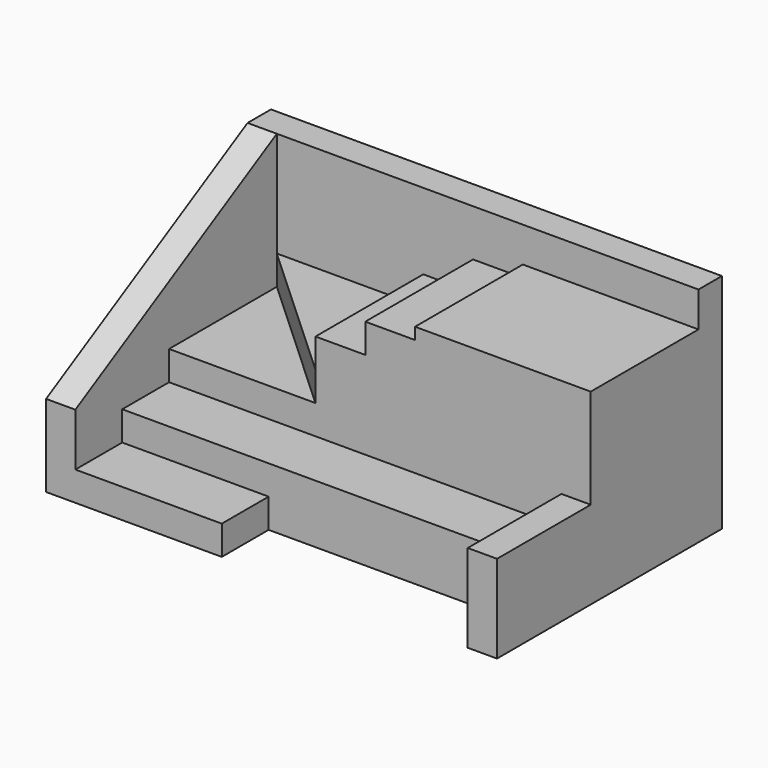
from build123d import *

# Parameters (mm, degrees)
F1_DEPTH  = 38
F3_DEPTH  = 25
F4_DEPTH  = 38
F0_W      = 25
F0_H      = 10
F5_DEPTH  = 5
F6_DEPTH  = 10
F7_DEPTH  = 15
F0_W_2    = 5
F0_H_2    = 5
F8_DEPTH  = 38
F0_H_3    = 23
F9_DEPTH  = 32
F11_DEPTH = 15
F12_DEPTH = 20
F0_W_3    = 8.5
F13_DEPTH = 25
F14_DEPTH = 30
F15_DEPTH = 32


# Not quite as in the source:
# - the program builds the solid bodies; features that only make, move or delete a surface that nothing else refers to are left out


with BuildPart() as f1:
    # F0 (on Top) → F1 (new body)
    with BuildSketch(Plane.XY):
        Polygon((-33.5, 19), (-38.5, 19), (-38.5, -24), (-33.5, -24), (-33.5, -14), (-33.5, -4), align=None)
    extrude(amount=F1_DEPTH)

    # F2 (on face) → F3 (cut)
    with BuildSketch(Plane.YZ.offset(-33.5)):
        Polygon((-24, 38), (-24, 14), (19, 38), align=None)
    extrude(amount=-F3_DEPTH, mode=Mode.SUBTRACT)

    # F0 (on Top) → F4 (join)
    with BuildSketch(Plane.XY):
        Polygon((33.5, 19), (33.5, 24), (-38.5, 24), (-38.5, 19), (-33.5, 19), (-8.5, 19), (0, 19), (8.5, 19), align=None)
    extrude(amount=F4_DEPTH)

    # F0 (on Top) → F5 (join)
    with BuildSketch(Plane.XY):
        with Locations((-21, -19)):
            Rectangle(F0_W, F0_H)
    extrude(amount=F5_DEPTH)

    # F0 (on Top) → F6 (join)
    with BuildSketch(Plane.XY):
        Polygon((33.5, -14), (33.5, -4), (8.5, -4), (0, -4), (-8.5, -4), (-33.5, -4), (-33.5, -14), (-8.5, -14), align=None)
    extrude(amount=F6_DEPTH)

    # F0 (on Top) → F7 (join)
    with BuildSketch(Plane.XY):
        Polygon((38.5, -24), (38.5, -4), (33.5, -4), (33.5, -14), (33.5, -24), align=None)
    extrude(amount=F7_DEPTH)

    # F0 (on Top) → F8 (join)
    with BuildSketch(Plane.XY):
        with Locations((36, 21.5)):
            Rectangle(F0_W_2, F0_H_2)
    extrude(amount=F8_DEPTH)

    # F0 (on Top) → F9 (join)
    with BuildSketch(Plane.XY):
        with Locations((36, 7.5)):
            Rectangle(F0_W_2, F0_H_3)
    extrude(amount=F9_DEPTH)

    # F0 (on Top) → F11 (join)
    with BuildSketch(Plane.XY):
        Polygon((-8.5, -4), (-33.5, 19), (-33.5, -4), align=None)
    extrude(amount=F11_DEPTH)

    # F0 (on Top) → F12 (join)
    with BuildSketch(Plane.XY):
        Polygon((-8.5, 19), (-33.5, 19), (-8.5, -4), align=None)
    extrude(amount=F12_DEPTH)

    # F0 (on Top) → F13 (join)
    with BuildSketch(Plane.XY):
        with Locations((-4.25, 7.5)):
            Rectangle(F0_W_3, F0_H_3)
    extrude(amount=F13_DEPTH)

    # F0 (on Top) → F14 (join)
    with BuildSketch(Plane.XY):
        with Locations((4.25, 7.5)):
            Rectangle(F0_W_3, F0_H_3)
    extrude(amount=F14_DEPTH)

    # F0 (on Top) → F15 (join)
    with BuildSketch(Plane.XY):
        with Locations((21, 7.5)):
            Rectangle(F0_W, F0_H_3)
    extrude(amount=F15_DEPTH)


solid = f1.part
